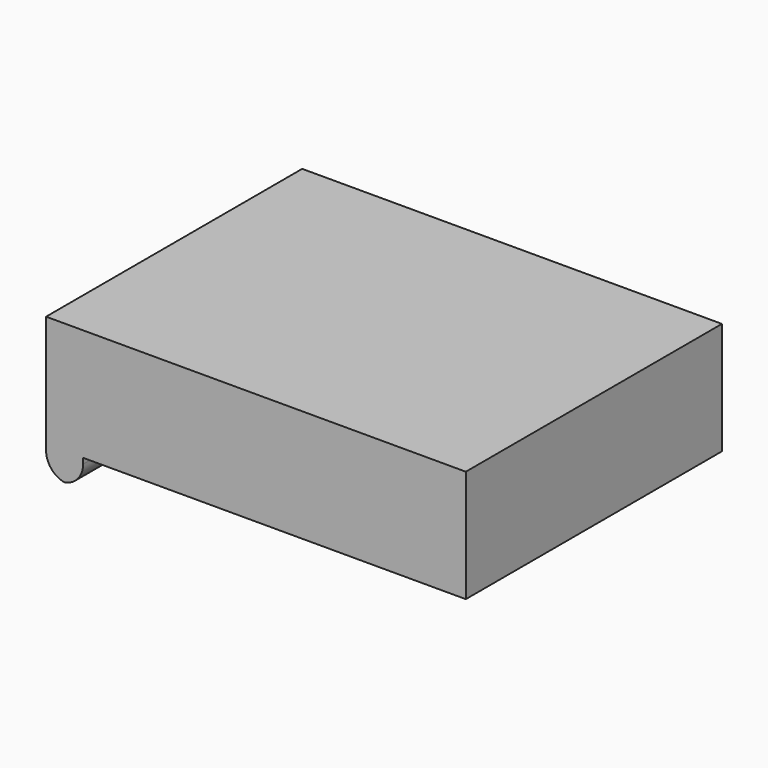
from build123d import *

# Parameters (mm, degrees)
F0_W        = 95.0071103871
F0_H        = 72.4661517888
F1_DEPTH    = 25.4
F2_W        = 8.3860605955
F2_H        = 72.4661517888
F3_DEPTH    = 6.35
F4_T1_DEPTH = 97.8661517888


# Not quite as in the source:
# - a fillet or chamfer that OpenCascade refuses, or shapes differently, is made with other operations: its cross-section is extruded or revolved along the edge and cut away or added


with BuildPart() as f1:
    # F0 (on Top) → F1 (new body)
    with BuildSketch(Plane.XY):
        with Locations((-23.8963868469, 6.1882724985)):
            Rectangle(F0_W, F0_H)
    extrude(amount=F1_DEPTH)

    # F2 (on face) → F3 (join)
    with BuildSketch(Plane(origin=(0, 0, 0), x_dir=(1, 0, 0), z_dir=(0, 0, -1))):
        with Locations((-67.2069117427, -6.1882724985)):
            Rectangle(F2_W, F2_H)
    extrude(amount=F3_DEPTH)

    # F4: fillet of radius 5.08 on 2 edges, made by hand

    # F4_s2 → F4_t1 (cut)
    with BuildSketch(Plane.XZ.offset(-55.121348393)):
        with BuildLine():
            ThreePointArc((-68.0938814449, -6.35), (-64.5017789965, -4.8621024484), (-63.0138814449, -1.27))
            Line((-63.0138814449, -1.27), (-63.0138814449, -6.35))
            Line((-63.0138814449, -6.35), (-68.0938814449, -6.35))
        make_face()
        with BuildLine():
            ThreePointArc((-71.3999420404, -1.27), (-69.9120444889, -4.8621024484), (-66.3199420404, -6.35))
            Line((-66.3199420404, -6.35), (-71.3999420404, -6.35))
            Line((-71.3999420404, -6.35), (-71.3999420404, -1.27))
        make_face()
    extrude(amount=F4_T1_DEPTH, mode=Mode.SUBTRACT)


solid = f1.part
